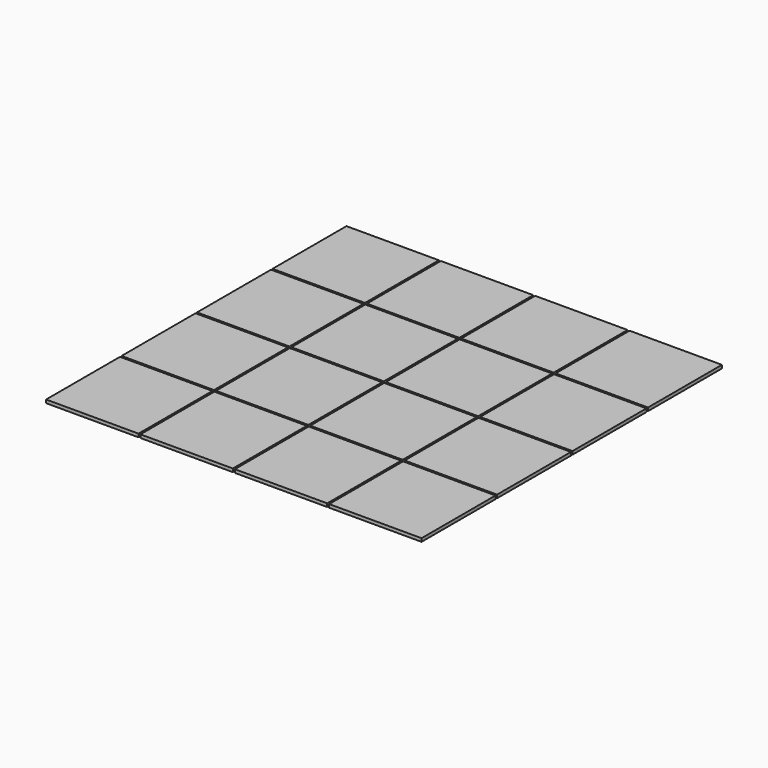
from build123d import *

# Parameters (mm, degrees)
F0_W     = 142
F0_H     = 142
F1_DEPTH = 5


# Not quite as in the source:
# - a feature names something its author has since deleted; it is built from what else it names


with BuildPart() as f1:
    # F0 (on Top) → F1 (new body)
    with BuildSketch(Plane.XY):
        with Locations((-219, -216)):
            Rectangle(F0_W, F0_H)
    extrude(amount=F1_DEPTH)


with BuildPart() as f1b:
    # F0 (on Top) → F1, piece 2 (new body)
    with BuildSketch(Plane.XY):
        with Locations((-219, -71)):
            Rectangle(F0_W, F0_H)
    extrude(amount=F1_DEPTH)


with BuildPart() as f1c:
    # F0 (on Top) → F1, piece 3 (new body)
    with BuildSketch(Plane.XY):
        with Locations((-219, 74)):
            Rectangle(F0_W, F0_H)
    extrude(amount=F1_DEPTH)


with BuildPart() as f1d:
    # F0 (on Top) → F1, piece 4 (new body)
    with BuildSketch(Plane.XY):
        with Locations((-219, 219)):
            Rectangle(F0_W, F0_H)
    extrude(amount=F1_DEPTH)


with BuildPart() as f1e:
    # F0 (on Top) → F1, piece 5 (new body)
    with BuildSketch(Plane.XY):
        with Locations((-74, 219)):
            Rectangle(F0_W, F0_H)
    extrude(amount=F1_DEPTH)


with BuildPart() as f1f:
    # F0 (on Top) → F1, piece 6 (new body)
    with BuildSketch(Plane.XY):
        with Locations((71, 219)):
            Rectangle(F0_W, F0_H)
    extrude(amount=F1_DEPTH)


with BuildPart() as f1g:
    # F0 (on Top) → F1, piece 7 (new body)
    with BuildSketch(Plane.XY):
        with Locations((216, 219)):
            Rectangle(F0_W, F0_H)
    extrude(amount=F1_DEPTH)


with BuildPart() as f1h:
    # F0 (on Top) → F1, piece 8 (new body)
    with BuildSketch(Plane.XY):
        with Locations((216, -71)):
            Rectangle(F0_W, F0_H)
    extrude(amount=F1_DEPTH)


with BuildPart() as f1i:
    # F0 (on Top) → F1, piece 9 (new body)
    with BuildSketch(Plane.XY):
        with Locations((71, -71)):
            Rectangle(F0_W, F0_H)
    extrude(amount=F1_DEPTH)


with BuildPart() as f1j:
    # F0 (on Top) → F1, piece 10 (new body)
    with BuildSketch(Plane.XY):
        with Locations((71, -216)):
            Rectangle(F0_W, F0_H)
    extrude(amount=F1_DEPTH)


with BuildPart() as f1k:
    # F0 (on Top) → F1, piece 11 (new body)
    with BuildSketch(Plane.XY):
        with Locations((216, -216)):
            Rectangle(F0_W, F0_H)
    extrude(amount=F1_DEPTH)


with BuildPart() as f1l:
    # F0 (on Top) → F1, piece 12 (new body)
    with BuildSketch(Plane.XY):
        with Locations((216, 74)):
            Rectangle(F0_W, F0_H)
    extrude(amount=F1_DEPTH)


with BuildPart() as f1m:
    # F0 (on Top) → F1, piece 13 (new body)
    with BuildSketch(Plane.XY):
        with Locations((71, 74)):
            Rectangle(F0_W, F0_H)
    extrude(amount=F1_DEPTH)


with BuildPart() as f1n:
    # F0 (on Top) → F1, piece 14 (new body)
    with BuildSketch(Plane.XY):
        with Locations((-74, 74)):
            Rectangle(F0_W, F0_H)
    extrude(amount=F1_DEPTH)


with BuildPart() as f1o:
    # F0 (on Top) → F1, piece 15 (new body)
    with BuildSketch(Plane.XY):
        with Locations((-74, -71)):
            Rectangle(F0_W, F0_H)
    extrude(amount=F1_DEPTH)


with BuildPart() as f1p:
    # F0 (on Top) → F1, piece 16 (new body)
    with BuildSketch(Plane.XY):
        with Locations((-74, -216)):
            Rectangle(F0_W, F0_H)
    extrude(amount=F1_DEPTH)


solid = Compound([f1.part, f1b.part, f1c.part, f1d.part, f1e.part, f1f.part, f1g.part, f1h.part, f1i.part, f1j.part, f1k.part, f1l.part, f1m.part, f1n.part, f1o.part, f1p.part])
